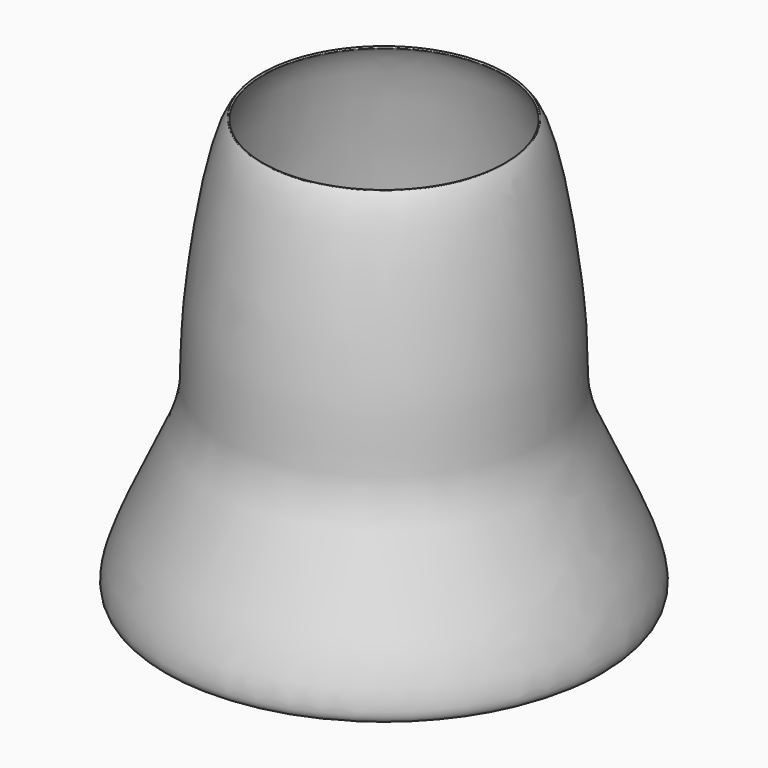
from build123d import *

# Parameters (mm, degrees)
F0_R        = 80
F0_R_2      = 15
F1_DEPTH    = 0.8
F4_T1_DEPTH = 0.8
F5_R        = 12
F6_R        = 0.35


# Not quite as in the source:
# - a fillet or chamfer that OpenCascade refuses, or shapes differently, is made with other operations: its cross-section is extruded or revolved along the edge and cut away or added
# - ends of sketch curves that miss each other by under 0.0002 mm in the source are joined
# - the dataset's text gives a spline's control points without its knots; the knots are read off the source's solid


with BuildPart() as f1:
    # F0 (on Top) → F1 (new body)
    with BuildSketch(Plane.XY):
        Circle(F0_R)
        with BuildLine():
            Line((-5, -24.4948974278), (-5, -25))
            Line((-5, -25), (-5, -69.8212002188))
            ThreePointArc((-5, -69.8212002188), (-23.9414100328, -65.778483455), (-41.0499801785, -56.700080488))
            Line((-41.0499801785, -56.700080488), (-12.2394680266, -22.3650491264))
            Line((-12.2394680266, -22.3650491264), (-11.9147943516, -21.9781181078))
            ThreePointArc((-11.9147943516, -21.9781181078), (-8.5505035831, -23.4923155196), (-5, -24.4948974278))
        make_face(mode=Mode.SUBTRACT)
        with BuildLine():
            Line((-67.8922184118, -17.0483629456), (-23.751952937, -9.2652432067))
            Line((-23.751952937, -9.2652432067), (-23.2545240078, -9.1775330655))
            ThreePointArc((-23.2545240078, -9.1775330655), (-21.6506350946, -12.5), (-19.5752387827, -15.5502420109))
            Line((-19.5752387827, -15.5502420109), (-19.8999124578, -15.9371730295))
            Line((-19.8999124578, -15.9371730295), (-48.7104246097, -50.2722043911))
            ThreePointArc((-48.7104246097, -50.2722043911), (-60.6217782649, -35), (-67.8922184118, -17.0483629456))
        make_face(mode=Mode.SUBTRACT)
        with BuildLine():
            Line((5, -25), (5, -24.4948974278))
            ThreePointArc((5, -24.4948974278), (8.5505035831, -23.4923155196), (11.9147943516, -21.9781181078))
            Line((11.9147943516, -21.9781181078), (12.2394680266, -22.3650491264))
            Line((12.2394680266, -22.3650491264), (41.0499801785, -56.700080488))
            ThreePointArc((41.0499801785, -56.700080488), (23.9414100328, -65.778483455), (5, -69.8212002188))
            Line((5, -69.8212002188), (5, -25))
        make_face(mode=Mode.SUBTRACT)
        with BuildLine():
            Line((48.7104246097, -50.2722043911), (19.8999124578, -15.9371730295))
            Line((19.8999124578, -15.9371730295), (19.5752387827, -15.5502420109))
            ThreePointArc((19.5752387827, -15.5502420109), (21.6506350946, -12.5), (23.2545240078, -9.1775330655))
            Line((23.2545240078, -9.1775330655), (23.751952937, -9.2652432067))
            Line((23.751952937, -9.2652432067), (67.8922184118, -17.0483629456))
            ThreePointArc((67.8922184118, -17.0483629456), (60.6217782649, -35), (48.7104246097, -50.2722043911))
        make_face(mode=Mode.SUBTRACT)
        with BuildLine():
            Line((-62.9669331122, 30.5804730905), (-24.1506350946, 8.1698729811))
            Line((-24.1506350946, 8.1698729811), (-23.7132034356, 7.917321695))
            ThreePointArc((-23.7132034356, 7.917321695), (-24.6201938253, 4.3412044417), (-24.9910057845, 0.6705444646))
            Line((-24.9910057845, 0.6705444646), (-25.4884347136, 0.5828343234))
            Line((-25.4884347136, 0.5828343234), (-69.6287001885, -7.2002854155))
            ThreePointArc((-69.6287001885, -7.2002854155), (-68.9365427109, 12.1553724367), (-62.9669331122, 30.5804730905))
        make_face(mode=Mode.SUBTRACT)
        with BuildLine():
            Line((-28.5787200099, 63.9003659034), (-13.2489666871, 21.782214803))
            Line((-13.2489666871, 21.782214803), (-13.0762114329, 21.3075736432))
            ThreePointArc((-13.0762114329, 21.3075736432), (-16.0696902422, 19.151111078), (-18.7132034356, 16.5775757328))
            Line((-18.7132034356, 16.5775757328), (-19.1506350946, 16.8301270189))
            Line((-19.1506350946, 16.8301270189), (-57.9669331122, 39.2407271283))
            ThreePointArc((-57.9669331122, 39.2407271283), (-44.9951326781, 53.6231110183), (-28.5787200099, 63.9003659034))
        make_face(mode=Mode.SUBTRACT)
        Circle(F0_R_2, mode=Mode.SUBTRACT)
        with BuildLine():
            Line((69.6287001885, -7.2002854155), (25.4884347136, 0.5828343234))
            Line((25.4884347136, 0.5828343234), (24.9910057845, 0.6705444646))
            ThreePointArc((24.9910057845, 0.6705444646), (24.6201938253, 4.3412044417), (23.7132034356, 7.917321695))
            Line((23.7132034356, 7.917321695), (24.1506350946, 8.1698729811))
            Line((24.1506350946, 8.1698729811), (62.9669331122, 30.5804730905))
            ThreePointArc((62.9669331122, 30.5804730905), (68.9365427109, 12.1553724367), (69.6287001885, -7.2002854155))
        make_face(mode=Mode.SUBTRACT)
        with BuildLine():
            Line((19.1817938021, 67.3205673367), (3.8520404792, 25.2024162363))
            Line((3.8520404792, 25.2024162363), (3.6792852251, 24.7277750765))
            ThreePointArc((3.6792852251, 24.7277750765), (0, 25), (-3.6792852251, 24.7277750765))
            Line((-3.6792852251, 24.7277750765), (-3.8520404792, 25.2024162363))
            Line((-3.8520404792, 25.2024162363), (-19.1817938021, 67.3205673367))
            ThreePointArc((-19.1817938021, 67.3205673367), (0, 70), (19.1817938021, 67.3205673367))
        make_face(mode=Mode.SUBTRACT)
        with BuildLine():
            Line((57.9669331122, 39.2407271283), (19.1506350946, 16.8301270189))
            Line((19.1506350946, 16.8301270189), (18.7132034356, 16.5775757328))
            ThreePointArc((18.7132034356, 16.5775757328), (16.0696902422, 19.151111078), (13.0762114329, 21.3075736432))
            Line((13.0762114329, 21.3075736432), (13.2489666871, 21.782214803))
            Line((13.2489666871, 21.782214803), (28.5787200099, 63.9003659034))
            ThreePointArc((28.5787200099, 63.9003659034), (44.9951326781, 53.6231110183), (57.9669331122, 39.2407271283))
        make_face(mode=Mode.SUBTRACT)
    extrude(amount=F1_DEPTH)

    # F2 (on Front) → F3 (revolve)
    with BuildSketch(Plane.XZ):
        with BuildLine():
            Line((79.9910168356, 0.7999495626), (80, 0))
            add(Edge.make_bspline(
                [(80, 0), (92.5339167711, 0.1407516681), (56.6350727896, 62.5998306003), (63.5471244419, 78.2826527399), (51.8772936907, 158.4757377507), (45, 160)],
                knots=[0, 0, 0, 0, 0.339080251, 0.6092942032, 1, 1, 1, 1], degree=3))
            Line((45, 160), (46.1887416489, 158.0775952356))
            add(Edge.make_bspline(
                [(79.9910168356, 0.7999495626), (80.5000040921, 0.8056653183), (81.1366015847, 0.911301472), (81.7674974777, 1.193589024), (82.154550482, 1.4698841236), (82.4772565163, 1.817868554), (82.8373336734, 2.3966491052), (83.1544632473, 3.3673460752), (83.2797885873, 4.9262210442), (83.1387550626, 6.8254880993), (82.7455480508, 9.0171377942), (81.9147235808, 12.2739372267), (80.3643651377, 16.8797482659), (77.8956966084, 22.9967414546), (75.0313449849, 29.4548022529), (71.9831703186, 36.0100880283), (68.9622940567, 42.4220778815), (66.6433910488, 47.4469358524), (65.0112665957, 51.1595720814), (63.9265611102, 53.7596370637), (62.9987244813, 56.1576953328), (61.9496294962, 59.1269962657), (60.9631767504, 62.4719113281), (60.2042151297, 66.1000246992), (59.7749836609, 69.5340832058), (59.5758835248, 72.9645144432), (59.5051009496, 76.5897684683), (59.4695826375, 79.9467121528), (59.406121129, 82.9400197099), (59.328768509, 85.3655742877), (59.2094283771, 87.997636962), (59.035757875, 90.8644965204), (58.8098414336, 93.9403316747), (58.4418859289, 98.2828009522), (57.8622719334, 104.0954236969), (56.9928292616, 111.4681529455), (55.9670987808, 119.0214908356), (54.8027699683, 126.5384998121), (53.5176770303, 133.8020124815), (52.1299239314, 140.5942240546), (50.6583804833, 146.6957811935), (49.3792386692, 151.0195769839), (48.337873441, 153.9060654672), (47.5532608346, 155.7534904638), (46.8311030494, 157.139493289), (46.3805915942, 157.8216988735), (46.1887416489, 158.0775952356)],
                knots=[0, 0, 0, 0, 0.015625, 0.0234375, 0.03125, 0.0390625, 0.046875, 0.0625, 0.078125, 0.09375, 0.109375, 0.125, 0.15625, 0.1875, 0.21875, 0.25, 0.28125, 0.3125, 0.328125, 0.34375, 0.359375, 0.375, 0.40625, 0.4375, 0.46875, 0.5, 0.53125, 0.5625, 0.578125, 0.59375, 0.609375, 0.625, 0.640625, 0.65625, 0.6875, 0.71875, 0.75, 0.78125, 0.8125, 0.84375, 0.875, 0.90625, 0.921875, 0.9375, 0.953125, 0.9652995174, 0.9652995174, 0.9652995174, 0.9652995174], degree=3))
        make_face()
    revolve(axis=Axis((0, 0, 10.9574086964), (0, 0, 1)))

    # F4: fillet of radius 6 on 18 edges, made by hand

    # F4_s2 → F4_t1 (join)
    with BuildSketch(Plane.XY):
        with BuildLine():
            ThreePointArc((-21.8195513821, -12.202752865), (-21.0827909776, -15.6952064295), (-22.4599770551, -18.9881392107))
            Line((-22.4599770551, -18.9881392107), (-19.5752387827, -15.5502420109))
            ThreePointArc((-19.5752387827, -15.5502420109), (-20.7649604886, -13.9217964324), (-21.8195513821, -12.202752865))
        make_face()
        with BuildLine():
            ThreePointArc((-8.8709677419, -23.3731883003), (-6.0616706495, -25.5749824869), (-5, -28.9827534924))
            Line((-5, -28.9827534924), (-5, -24.4948974278))
            ThreePointArc((-5, -24.4948974278), (-6.9581243425, -24.012174113), (-8.8709677419, -23.3731883003))
        make_face()
        with BuildLine():
            ThreePointArc((8.2284402945, -23.6070491659), (11.7957727435, -23.4879400044), (14.7995326239, -25.4160153076))
            Line((14.7995326239, -25.4160153076), (11.9147943516, -21.9781181078))
            ThreePointArc((11.9147943516, -21.9781181078), (10.1044955144, -22.8669886605), (8.2284402945, -23.6070491659))
        make_face()
        with BuildLine():
            ThreePointArc((21.4776696682, -12.7949093636), (24.1338429743, -10.4106293545), (27.6741994546, -9.9568410928))
            Line((27.6741994546, -9.9568410928), (23.2545240078, -9.1775330655))
            ThreePointArc((23.2545240078, -9.1775330655), (22.4391096211, -11.0220850755), (21.4776696682, -12.7949093636))
        make_face()
        with BuildLine():
            ThreePointArc((24.6772587065, 4.0041107295), (25.1794198597, 7.5379304716), (27.599800796, 10.1612497273))
            Line((27.599800796, 10.1612497273), (23.7132034356, 7.917321695))
            ThreePointArc((23.7132034356, 7.917321695), (24.2742149532, 5.9801746132), (24.6772587065, 4.0041107295))
        make_face()
        with BuildLine():
            ThreePointArc((16.3300841388, 18.9295629115), (14.4432663547, 21.9594088553), (14.6111486074, 25.5247788702))
            Line((14.6111486074, 25.5247788702), (13.0762114329, 21.3075736432))
            ThreePointArc((13.0762114329, 21.3075736432), (14.7511453309, 20.1842441381), (16.3300841388, 18.9295629115))
        make_face()
        with BuildLine():
            ThreePointArc((22.599800796, 18.8215037651), (19.1177492103, 18.0370520153), (15.8062909645, 19.3690775708))
            ThreePointArc((15.8062909645, 19.3690775708), (17.3160906107, 18.0319994998), (18.7132034356, 16.5775757328))
            Line((18.7132034356, 16.5775757328), (22.599800796, 18.8215037651))
        make_face()
        with BuildLine():
            ThreePointArc((29.4106812313, -0.1087635627), (26.2390390981, 1.5285311491), (24.5585244333, 4.6774862544))
            ThreePointArc((24.5585244333, 4.6774862544), (24.8556408452, 2.6827445224), (24.9910057845, 0.6705444646))
            Line((24.9910057845, 0.6705444646), (29.4106812313, -0.1087635627))
        make_face()
        with BuildLine():
            ThreePointArc((22.4599770551, -18.9881392107), (21.0827909776, -15.6952064295), (21.8195513821, -12.202752865))
            ThreePointArc((21.8195513821, -12.202752865), (20.7649604886, -13.9217964324), (19.5752387827, -15.5502420109))
            Line((19.5752387827, -15.5502420109), (22.4599770551, -18.9881392107))
        make_face()
        with BuildLine():
            ThreePointArc((5, -28.9827534924), (6.0616706495, -25.5749824869), (8.8709677419, -23.3731883003))
            ThreePointArc((8.8709677419, -23.3731883003), (6.9581243425, -24.012174113), (5, -24.4948974278))
            Line((5, -24.4948974278), (5, -28.9827534924))
        make_face()
        with BuildLine():
            ThreePointArc((-8.2284402945, -23.6070491659), (-11.7957727435, -23.4879400044), (-14.7995326239, -25.4160153076))
            Line((-14.7995326239, -25.4160153076), (-11.9147943516, -21.9781181078))
            ThreePointArc((-11.9147943516, -21.9781181078), (-10.1044955144, -22.8669886605), (-8.2284402945, -23.6070491659))
        make_face()
        with BuildLine():
            ThreePointArc((-27.6741994546, -9.9568410928), (-24.1338429743, -10.4106293545), (-21.4776696682, -12.7949093636))
            ThreePointArc((-21.4776696682, -12.7949093636), (-22.4391096211, -11.0220850755), (-23.2545240078, -9.1775330655))
            Line((-23.2545240078, -9.1775330655), (-27.6741994546, -9.9568410928))
        make_face()
        with BuildLine():
            ThreePointArc((-24.5585244333, 4.6774862544), (-26.2390390981, 1.5285311491), (-29.4106812313, -0.1087635627))
            Line((-29.4106812313, -0.1087635627), (-24.9910057845, 0.6705444646))
            ThreePointArc((-24.9910057845, 0.6705444646), (-24.8556408452, 2.6827445224), (-24.5585244333, 4.6774862544))
        make_face()
        with BuildLine():
            ThreePointArc((-27.599800796, 10.1612497273), (-25.1794198597, 7.5379304716), (-24.6772587065, 4.0041107295))
            ThreePointArc((-24.6772587065, 4.0041107295), (-24.2742149532, 5.9801746132), (-23.7132034356, 7.917321695))
            Line((-23.7132034356, 7.917321695), (-27.599800796, 10.1612497273))
        make_face()
        with BuildLine():
            ThreePointArc((-15.8062909645, 19.3690775708), (-19.1177492103, 18.0370520153), (-22.599800796, 18.8215037651))
            Line((-22.599800796, 18.8215037651), (-18.7132034356, 16.5775757328))
            ThreePointArc((-18.7132034356, 16.5775757328), (-17.3160906107, 18.0319994998), (-15.8062909645, 19.3690775708))
        make_face()
        with BuildLine():
            ThreePointArc((-14.6111486074, 25.5247788702), (-14.4432663547, 21.9594088553), (-16.3300841388, 18.9295629115))
            ThreePointArc((-16.3300841388, 18.9295629115), (-14.7511453309, 20.1842441381), (-13.0762114329, 21.3075736432))
            Line((-13.0762114329, 21.3075736432), (-14.6111486074, 25.5247788702))
        make_face()
        with BuildLine():
            ThreePointArc((5.2142223995, 28.9449803035), (3.0510519968, 26.105835784), (-0.3418817139, 24.9976622286))
            ThreePointArc((-0.3418817139, 24.9976622286), (1.6741491325, 24.9438815079), (3.6792852251, 24.7277750765))
            Line((3.6792852251, 24.7277750765), (5.2142223995, 28.9449803035))
        make_face()
        with BuildLine():
            ThreePointArc((0.3418817139, 24.9976622286), (-3.0510519968, 26.105835784), (-5.2142223995, 28.9449803035))
            Line((-5.2142223995, 28.9449803035), (-3.6792852251, 24.7277750765))
            ThreePointArc((-3.6792852251, 24.7277750765), (-1.6741491325, 24.9438815079), (0.3418817139, 24.9976622286))
        make_face()
    extrude(amount=F4_T1_DEPTH)

    # F5
    f5_edges = [f1.edges().sort_by_distance(p)[0] for p in [
        (-69.6287, -7.200285, 0.4),
        (-67.892218, -17.048363, 0.4),
        (-48.710425, -50.272204, 0.4),
        (-41.04998, -56.70008, 0.4),
        (-5, -69.8212, 0.4),
        (5, -69.8212, 0.4),
        (41.04998, -56.70008, 0.4),
        (48.710425, -50.272204, 0.4),
        (67.892218, -17.048363, 0.4),
        (69.6287, -7.200285, 0.4),
        (62.966933, 30.580473, 0.4),
        (57.966933, 39.240727, 0.4),
        (28.57872, 63.900366, 0.4),
        (19.181794, 67.320567, 0.4),
        (-19.181794, 67.320567, 0.4),
        (-28.57872, 63.900366, 0.4),
        (-57.966933, 39.240727, 0.4),
        (-62.966933, 30.580473, 0.4),
    ]]
    fillet(f5_edges, radius=F5_R)

    # F6
    f6_edges = [f1.edges().sort_by_distance(p)[0] for p in [
        (-45, 0, 160),
        (-46.188742, 0, 158.077595),
    ]]
    fillet(f6_edges, radius=F6_R)


solid = f1.part
